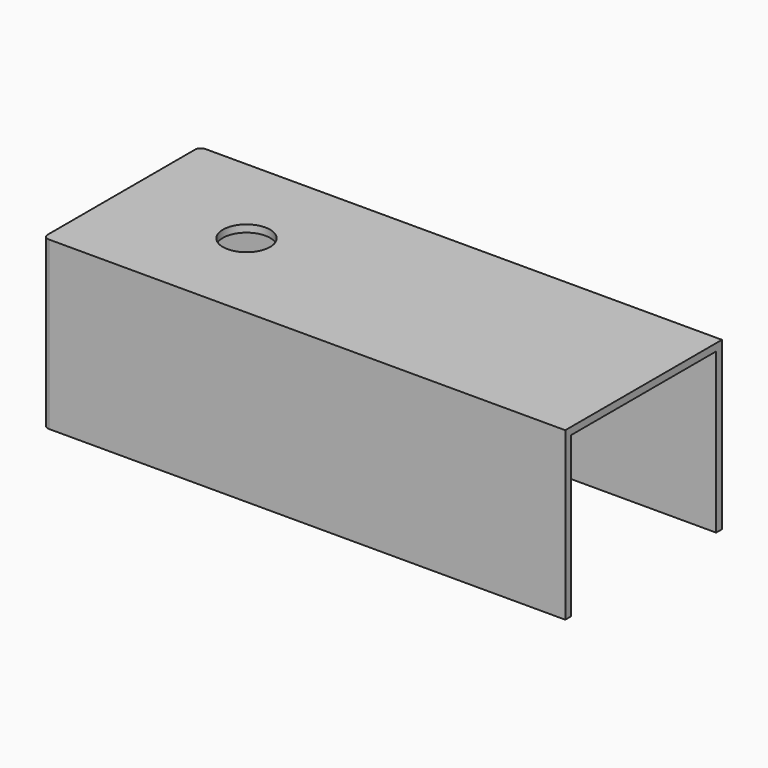
from build123d import *

# Parameters (mm, degrees)
F0_W     = 72
F0_H     = 24
F1_DEPTH = 27
F2_T     = -1
F3_R     = 3.25
F4_DEPTH = 25
F5_W     = 72
F5_H     = 27
F5_R     = 3.25
F6_DEPTH = 1
F8_DEPTH = 1
F9_R     = 0.8


# Not quite as in the source:
# - a feature names something its author has since deleted; it is built from what else it names


with BuildPart() as f1:
    # F0 (on Front) → F1 (new body)
    with BuildSketch(Plane.XZ):
        Rectangle(F0_W, F0_H)
    extrude(amount=F1_DEPTH)

    # F2
    f2_openings = [f1.faces().sort_by_distance(p)[0] for p in [
        (36, -13.5, 0),
    ]]
    offset(amount=F2_T, openings=f2_openings)

    # F3 (on face) → F4 (cut)
    with BuildSketch(Plane.XY.offset(12)):
        with Locations((-18.75, -13.5)):
            Circle(F3_R)
    extrude(amount=-F4_DEPTH, mode=Mode.SUBTRACT)

    # F5 (on face) → F6 (cut)
    with BuildSketch(Plane(origin=(0, 0, -12), x_dir=(1, 0, 0), z_dir=(0, 0, -1))):
        with Locations((0, 13.5)):
            Rectangle(F5_W, F5_H)
        with Locations((-18.75, 13.5)):
            Circle(F5_R, mode=Mode.SUBTRACT)
    extrude(amount=-F6_DEPTH, mode=Mode.SUBTRACT)

    # F9
    f9_edges = [f1.edges().sort_by_distance(p)[0] for p in [
        (-36, -27, 0.5),
        (-36, 0, 0.5),
    ]]
    fillet(f9_edges, radius=F9_R)


with BuildPart() as f8:
    # F7 (on face) → F8 (new body)
    with BuildSketch(Plane.XY.offset(12)):
        with BuildLine():
            Line((-36, -1), (-36, -27))
            Line((-36, -27), (36, -27))
            Line((36, -27), (36, -16.75))
            Line((36, -16.75), (-18.75, -16.75))
            ThreePointArc((-18.75, -16.75), (-22, -13.5), (-18.75, -10.25))
            Line((-18.75, -10.25), (36, -10.25))
            Line((36, -10.25), (36, -1))
            Line((36, -1), (-36, -1))
        make_face()
    extrude(amount=F8_DEPTH)


solid = f1.part
